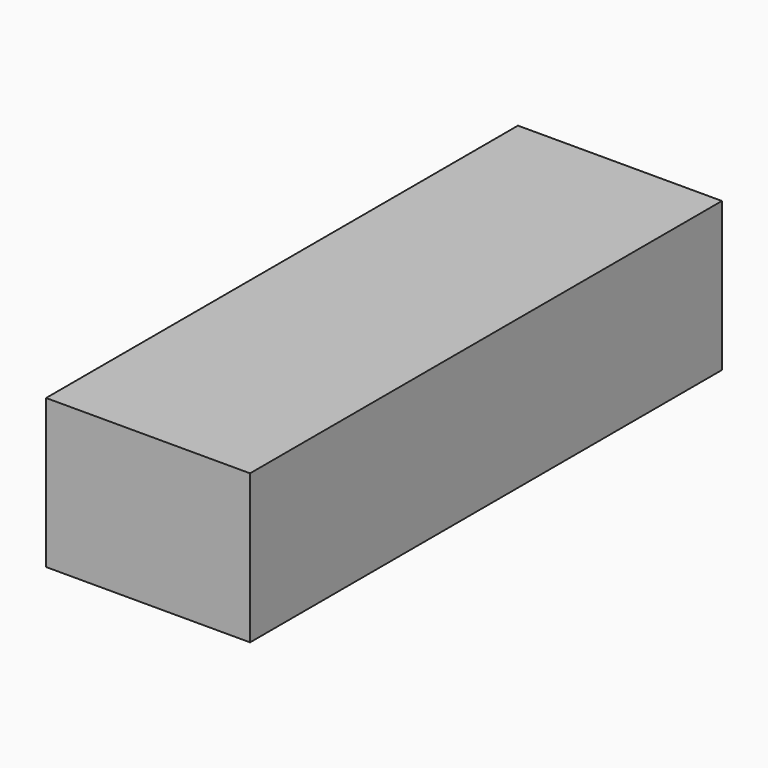
from build123d import *

# Parameters (mm, degrees)
F0_W     = 107
F0_H     = 27
F1_DEPTH = 18.5


with BuildPart() as f1:
    # F0 (on Right) → F1 (new body, symmetric)
    with BuildSketch(Plane.YZ):
        Rectangle(F0_W, F0_H)
    extrude(amount=F1_DEPTH, both=True)


solid = f1.part
